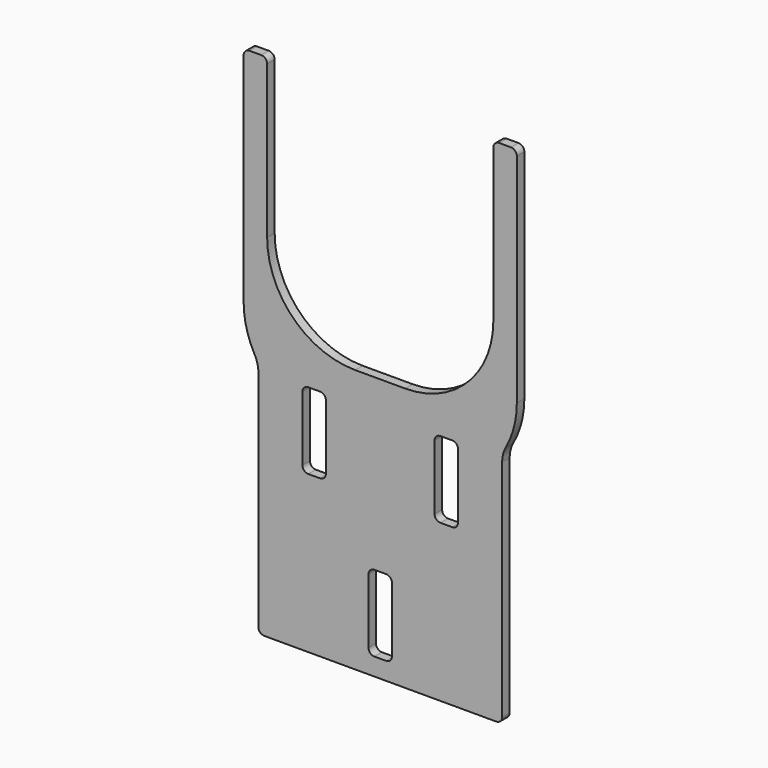
from build123d import *

# Parameters (mm, degrees)
F0_W     = 4
F0_H     = 13
F1_DEPTH = 1.6
F2_R     = 15
F3_R     = 5
F4_R     = 1


# Not quite as in the source:
# - a feature names something its author has since deleted; it is built from what else it names


with BuildPart() as f1:
    # F0 (on Front) → F1 (new body)
    with BuildSketch(Plane.XZ):
        Polygon((-19.25, 42), (-23.25, 42), (-23.25, 0), (-20.75, -4.3301270189), (-20.75, -44.8660254038), (20.75, -44.8660254038), (20.75, -4.3301270189), (23.25, 0), (23.25, 42), (19.25, 42), (19.25, 0), (-19.25, 0), align=None)
        with Locations((-11.25, -11.6689147807)):
            Rectangle(F0_W, F0_H, mode=Mode.SUBTRACT)
        with Locations((0, -35.3660254038)):
            Rectangle(F0_W, F0_H, mode=Mode.SUBTRACT)
        with Locations((11.25, -11.6689147807)):
            Rectangle(F0_W, F0_H, mode=Mode.SUBTRACT)
    extrude(amount=F1_DEPTH)

    # F2
    f2_edges = [f1.edges().sort_by_distance(p)[0] for p in [
        (-19.25, -0.8, 0),
        (19.25, -0.8, 0),
        (23.25, -0.8, 0),
        (-23.25, -0.8, 0),
    ]]
    fillet(f2_edges, radius=F2_R)

    # F3
    f3_edges = [f1.edges().sort_by_distance(p)[0] for p in [
        (-20.75, -0.8, -4.330127),
        (20.75, -0.8, -4.330127),
    ]]
    fillet(f3_edges, radius=F3_R)

    # F4
    f4_edges = [f1.edges().sort_by_distance(p)[0] for p in [
        (-13.25, -0.8, -5.168915),
        (-13.25, -0.8, -18.168915),
        (-9.25, -0.8, -5.168915),
        (-9.25, -0.8, -18.168915),
        (13.25, -0.8, -18.168915),
        (13.25, -0.8, -5.168915),
        (9.25, -0.8, -5.168915),
        (9.25, -0.8, -18.168915),
        (-2, -0.8, -41.866025),
        (-2, -0.8, -28.866025),
        (2, -0.8, -28.866025),
        (2, -0.8, -41.866025),
        (20.75, -0.8, -44.866025),
        (-20.75, -0.8, -44.866025),
        (-19.25, -0.8, 42),
        (-23.25, -0.8, 42),
        (19.25, -0.8, 42),
        (23.25, -0.8, 42),
    ]]
    fillet(f4_edges, radius=F4_R)


solid = f1.part
